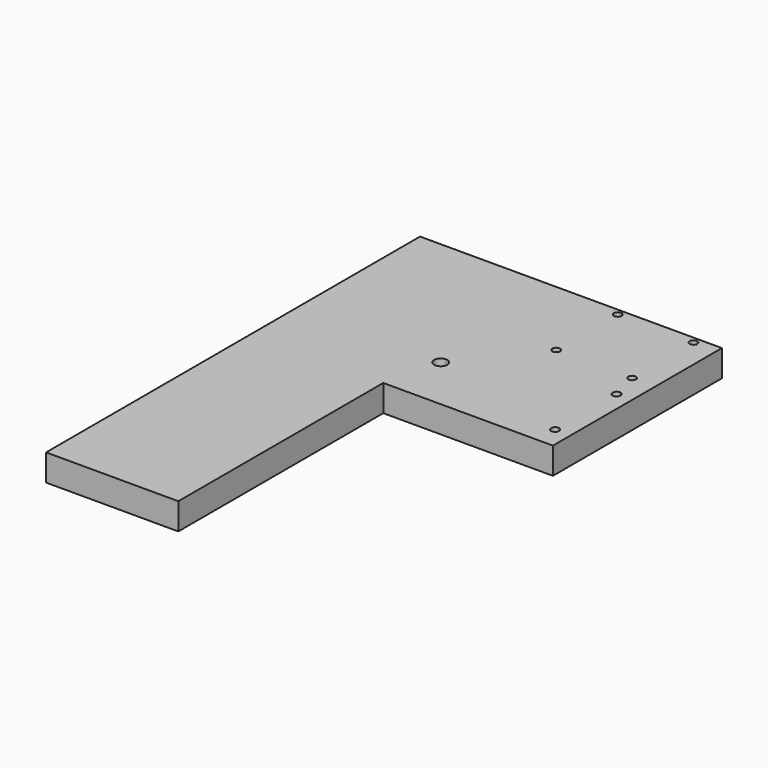
from build123d import *

# Parameters (mm, degrees)
F0_W     = 39.75
F0_H     = 5
F0_W_2   = 4
F0_H_2   = 9
F0_H_3   = 77
F0_W_3   = 3
F0_H_4   = 26.5
F0_H_5   = 1.95
F0_W_4   = 5
F0_H_6   = 17
F0_H_7   = 23.1
F1_DEPTH = 8


with BuildPart() as f1:
    # F0 (on Top) → F1 (new body)
    with BuildSketch(Plane.XY):
        Polygon((-32.4509056807, -49.8260023594), (-32.4509056807, -58.8260023594), (7.2990943193, -58.8260023594), (7.2990943193, -49.8260023594), (-26.0348562151, -49.8260023594), align=None)
        with Locations((-12.5759056807, -61.3260023594)):
            Rectangle(F0_W, F0_H)
        with Locations((9.2990943193, -54.3260023594)):
            Rectangle(F0_W_2, F0_H_2)
        Polygon((11.2990943193, -58.8260023594), (7.2990943193, -58.8260023594), (7.2990943193, -63.8260023594), (14.2990943193, -63.8260023594), (19.2990943193, -63.8260023594), (58.2990943193, -63.8260023594), (58.2990943193, -22.3260023594), (53.2990943193, -22.3260023594), (53.2990943193, -25.3760023594), (53.2990943193, -27.3260023594), (51.3490943193, -27.3260023594), (28.5490943193, -27.3260023594), (23.2990943193, -27.3260023594), (23.2990943193, -32.3260023594), (53.5990943193, -32.3260023594), (55.2990943193, -32.3260023594), (55.2990943193, -34.0260023594), (55.2990943193, -57.1260023594), (55.2990943193, -58.8260023594), (53.5990943193, -58.8260023594), (23.2990943193, -58.8260023594), (19.2990943193, -58.8260023594), (14.2990943193, -58.8260023594), align=None)
        with BuildLine():
            Line((-32.4509056807, -0.3260023594), (-32.4509056807, -49.8260023594))
            Line((-32.4509056807, -49.8260023594), (-26.0348562151, -49.8260023594))
            Line((-26.0348562151, -49.8260023594), (7.2990943193, -49.8260023594))
            Line((7.2990943193, -49.8260023594), (11.2990943193, -49.8260023594))
            Line((11.2990943193, -49.8260023594), (11.2990943193, -49.2260023594))
            ThreePointArc((11.2990943193, -49.2260023594), (9.2990943193, -47.2260023594), (11.2990943193, -45.2260023594))
            Line((11.2990943193, -45.2260023594), (11.2990943193, -0.3260023594))
            Line((11.2990943193, -0.3260023594), (-32.4509056807, -0.3260023594))
        make_face()
        with Locations((-12.5759056807, -102.3260023594)):
            Rectangle(F0_W, F0_H_3)
        with Locations((12.7990943193, -54.3260023594)):
            Rectangle(F0_W_3, F0_H_2)
        Polygon((14.2990943193, -49.8260023594), (14.2990943193, -58.8260023594), (19.2990943193, -58.8260023594), (19.2990943193, -32.3260023594), (23.2990943193, -32.3260023594), (23.2990943193, -27.3260023594), (19.2990943193, -27.3260023594), (19.2990943193, -25.3760023594), (19.2990943193, -2.2760023594), (19.2990943193, -0.3260023594), (14.2990943193, -0.3260023594), (14.2990943193, -27.3260023594), (14.2990943193, -32.3260023594), (14.2990943193, -47.2260023594), align=None)
        with BuildLine():
            Line((11.2990943193, -49.2260023594), (11.2990943193, -49.8260023594))
            Line((11.2990943193, -49.8260023594), (14.2990943193, -49.8260023594))
            Line((14.2990943193, -49.8260023594), (14.2990943193, -47.2260023594))
            Line((14.2990943193, -47.2260023594), (13.2990943193, -47.2260023594))
            ThreePointArc((13.2990943193, -47.2260023594), (12.7133078817, -48.6402159218), (11.2990943193, -49.2260023594))
        make_face()
        with BuildLine():
            Line((14.2990943193, -0.3260023594), (11.2990943193, -0.3260023594))
            Line((11.2990943193, -0.3260023594), (11.2990943193, -45.2260023594))
            ThreePointArc((11.2990943193, -45.2260023594), (12.7133078817, -45.811788797), (13.2990943193, -47.2260023594))
            Line((13.2990943193, -47.2260023594), (14.2990943193, -47.2260023594))
            Line((14.2990943193, -47.2260023594), (14.2990943193, -32.3260023594))
            Line((14.2990943193, -32.3260023594), (14.2990943193, -27.3260023594))
            Line((14.2990943193, -27.3260023594), (14.2990943193, -0.3260023594))
        make_face()
        with Locations((21.2990943193, -45.5760023594)):
            Rectangle(F0_W_2, F0_H_4)
        with BuildLine():
            Line((23.2990943193, -32.3260023594), (23.2990943193, -58.8260023594))
            Line((23.2990943193, -58.8260023594), (53.5990943193, -58.8260023594))
            Line((53.5990943193, -58.8260023594), (53.5990943193, -58.3260023594))
            ThreePointArc((53.5990943193, -58.3260023594), (52.7505661819, -56.277474222), (54.7990943193, -57.1260023594))
            Line((54.7990943193, -57.1260023594), (55.2990943193, -57.1260023594))
            Line((55.2990943193, -57.1260023594), (55.2990943193, -34.0260023594))
            Line((55.2990943193, -34.0260023594), (54.7990943193, -34.0260023594))
            ThreePointArc((54.7990943193, -34.0260023594), (52.7505661819, -34.8745304968), (53.5990943193, -32.8260023594))
            Line((53.5990943193, -32.8260023594), (53.5990943193, -32.3260023594))
            Line((53.5990943193, -32.3260023594), (23.2990943193, -32.3260023594))
        make_face()
        with Locations((21.2990943193, -1.3010023594)):
            Rectangle(F0_W_2, F0_H_5)
        with BuildLine():
            Line((53.5990943193, -58.3260023594), (53.5990943193, -58.8260023594))
            Line((53.5990943193, -58.8260023594), (55.2990943193, -58.8260023594))
            Line((55.2990943193, -58.8260023594), (55.2990943193, -57.1260023594))
            Line((55.2990943193, -57.1260023594), (54.7990943193, -57.1260023594))
            ThreePointArc((54.7990943193, -57.1260023594), (54.4476224568, -57.9745304968), (53.5990943193, -58.3260023594))
        make_face()
        with Locations((55.7990943193, -13.8260023594)):
            Rectangle(F0_W_4, F0_H_6)
        with BuildLine():
            Line((28.5490943193, -0.3260023594), (23.2990943193, -0.3260023594))
            Line((23.2990943193, -0.3260023594), (23.2990943193, -2.2760023594))
            Line((23.2990943193, -2.2760023594), (27.3990943193, -2.2760023594))
            ThreePointArc((27.3990943193, -2.2760023594), (27.735921521, -1.462829561), (28.5490943193, -1.1260023594))
            Line((28.5490943193, -1.1260023594), (28.5490943193, -0.3260023594))
        make_face()
        with Locations((21.2990943193, -13.8260023594)):
            Rectangle(F0_W_2, F0_H_7)
        with BuildLine():
            Line((55.2990943193, -32.3260023594), (53.5990943193, -32.3260023594))
            Line((53.5990943193, -32.3260023594), (53.5990943193, -32.8260023594))
            ThreePointArc((53.5990943193, -32.8260023594), (54.4476224568, -33.177474222), (54.7990943193, -34.0260023594))
            Line((54.7990943193, -34.0260023594), (55.2990943193, -34.0260023594))
            Line((55.2990943193, -34.0260023594), (55.2990943193, -32.3260023594))
        make_face()
        with BuildLine():
            Line((23.2990943193, -25.3760023594), (23.2990943193, -27.3260023594))
            Line((23.2990943193, -27.3260023594), (28.5490943193, -27.3260023594))
            Line((28.5490943193, -27.3260023594), (28.5490943193, -26.5260023594))
            ThreePointArc((28.5490943193, -26.5260023594), (27.735921521, -26.1891751578), (27.3990943193, -25.3760023594))
            Line((27.3990943193, -25.3760023594), (23.2990943193, -25.3760023594))
        make_face()
        with Locations((21.2990943193, -26.3510023594)):
            Rectangle(F0_W_2, F0_H_5)
        with BuildLine():
            Line((53.2990943193, -25.3760023594), (53.2990943193, -22.3260023594))
            Line((53.2990943193, -22.3260023594), (53.2990943193, -5.3260023594))
            Line((53.2990943193, -5.3260023594), (53.2990943193, -2.2760023594))
            Line((53.2990943193, -2.2760023594), (52.4990943193, -2.2760023594))
            ThreePointArc((52.4990943193, -2.2760023594), (50.535921521, -3.0891751578), (51.3490943193, -1.1260023594))
            Line((51.3490943193, -1.1260023594), (51.3490943193, -0.3260023594))
            Line((51.3490943193, -0.3260023594), (28.5490943193, -0.3260023594))
            Line((28.5490943193, -0.3260023594), (28.5490943193, -1.1260023594))
            ThreePointArc((28.5490943193, -1.1260023594), (29.3622671177, -1.462829561), (29.6990943193, -2.2760023594))
            ThreePointArc((29.6990943193, -2.2760023594), (28.5490943193, -3.4260023594), (27.3990943193, -2.2760023594))
            Line((27.3990943193, -2.2760023594), (23.2990943193, -2.2760023594))
            Line((23.2990943193, -2.2760023594), (23.2990943193, -25.3760023594))
            Line((23.2990943193, -25.3760023594), (27.3990943193, -25.3760023594))
            ThreePointArc((27.3990943193, -25.3760023594), (28.5490943193, -24.2260023594), (29.6990943193, -25.3760023594))
            ThreePointArc((29.6990943193, -25.3760023594), (29.3622671177, -26.1891751578), (28.5490943193, -26.5260023594))
            Line((28.5490943193, -26.5260023594), (28.5490943193, -27.3260023594))
            Line((28.5490943193, -27.3260023594), (51.3490943193, -27.3260023594))
            Line((51.3490943193, -27.3260023594), (51.3490943193, -26.5260023594))
            ThreePointArc((51.3490943193, -26.5260023594), (50.535921521, -24.562829561), (52.4990943193, -25.3760023594))
            Line((52.4990943193, -25.3760023594), (53.2990943193, -25.3760023594))
        make_face()
        Polygon((53.2990943193, -5.3260023594), (58.2990943193, -5.3260023594), (58.2990943193, -0.3260023594), (53.2990943193, -0.3260023594), (53.2990943193, -2.2760023594), align=None)
        with BuildLine():
            Line((53.2990943193, -27.3260023594), (53.2990943193, -25.3760023594))
            Line((53.2990943193, -25.3760023594), (52.4990943193, -25.3760023594))
            ThreePointArc((52.4990943193, -25.3760023594), (52.1622671177, -26.1891751578), (51.3490943193, -26.5260023594))
            Line((51.3490943193, -26.5260023594), (51.3490943193, -27.3260023594))
            Line((51.3490943193, -27.3260023594), (53.2990943193, -27.3260023594))
        make_face()
        with BuildLine():
            Line((53.2990943193, -0.3260023594), (51.3490943193, -0.3260023594))
            Line((51.3490943193, -0.3260023594), (51.3490943193, -1.1260023594))
            ThreePointArc((51.3490943193, -1.1260023594), (52.1622671177, -1.462829561), (52.4990943193, -2.2760023594))
            Line((52.4990943193, -2.2760023594), (53.2990943193, -2.2760023594))
            Line((53.2990943193, -2.2760023594), (53.2990943193, -0.3260023594))
        make_face()
    extrude(amount=F1_DEPTH)


solid = f1.part
